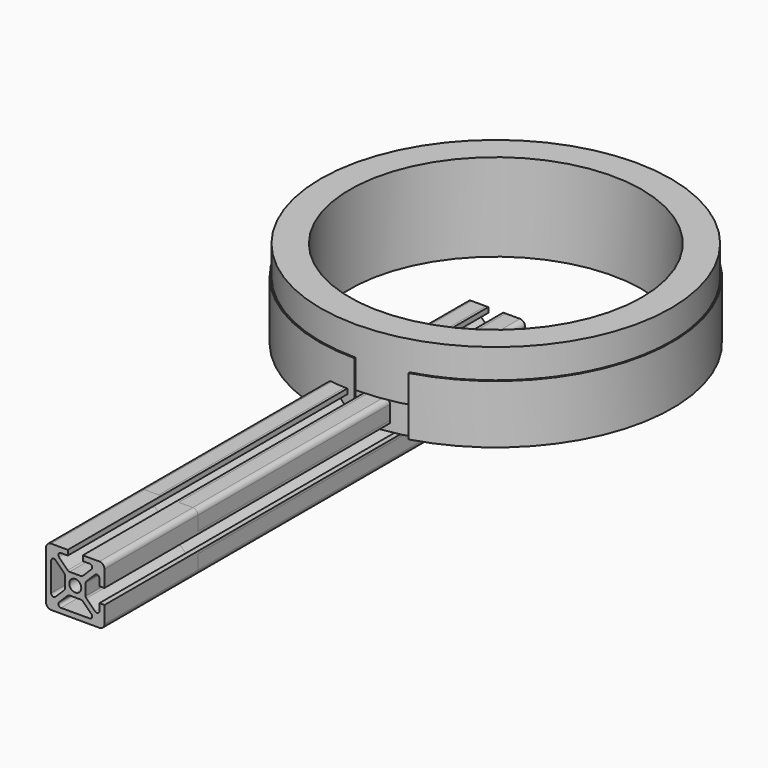
from build123d import *

# Parameters (mm, degrees)
F0_R      = 2.6035
F1_DEPTH  = 228.6
F2_R      = 2.6035
F3_DEPTH  = 177.8
F4_DEPTH  = 228.601
F0_W      = 6.5024
F0_H      = 2.2098
F0_H_2    = 2.1024142881
F0_H_3    = 4.3122142881
F5_DEPTH  = 228.601
F0_W_2    = 4.9525789589
F0_H_4    = 6.5024
F0_W_3    = 2.2098
F0_W_4    = 2.7427789589
F6_DEPTH  = 228.601
F7_R      = 1.10489
F8_R      = 76.2
F8_R_2    = 63.5
F9_DEPTH  = 38.1
F10_R     = 76.2
F10_R_2   = 74.6125
F11_DEPTH = 12.954
F13_DEPTH = 25.4


# Not quite as in the source:
# - a fillet or chamfer is up to 0.001 mm smaller than in the source, because OpenCascade refuses the exact size


with BuildPart() as f1:
    # F0 (on Front) → F1 (new body)
    with BuildSketch(Plane.XZ):
        with BuildLine():
            ThreePointArc((12.7, 10.4902), (12.0527645651, 12.0527645651), (10.4902, 12.7))
            Line((10.4902, 12.7), (3.2512, 12.7))
            Line((3.2512, 12.7), (3.2512, 10.4902))
            Line((3.2512, 10.4902), (6.2601708699, 10.4902))
            ThreePointArc((6.2601708699, 10.4902), (7.2809653653, 9.8081269244), (7.0414531524, 8.6040177175))
            Line((7.0414531524, 8.6040177175), (3.2822531524, 4.8448177175))
            ThreePointArc((3.2822531524, 4.8448177175), (2.9237977943, 4.6053055045), (2.5009708699, 4.5212))
            Line((2.5009708699, 4.5212), (-2.5009708699, 4.5212))
            ThreePointArc((-2.5009708699, 4.5212), (-2.9237977943, 4.6053055045), (-3.2822531524, 4.8448177175))
            Line((-3.2822531524, 4.8448177175), (-7.0414531524, 8.6040177175))
            ThreePointArc((-7.0414531524, 8.6040177175), (-7.2809653653, 9.8081269244), (-6.2601708699, 10.4902))
            Line((-6.2601708699, 10.4902), (-3.2512, 10.4902))
            Line((-3.2512, 10.4902), (-3.2512, 12.7))
            Line((-3.2512, 12.7), (-10.4902, 12.7))
            ThreePointArc((-10.4902, 12.7), (-12.0527645651, 12.0527645651), (-12.7, 10.4902))
            Line((-12.7, 10.4902), (-12.7, -10.4902))
            ThreePointArc((-12.7, -10.4902), (-12.0527645651, -12.0527645651), (-10.4902, -12.7))
            Line((-10.4902, -12.7), (10.4902, -12.7))
            ThreePointArc((10.4902, -12.7), (12.0527645651, -12.0527645651), (12.7, -10.4902))
            Line((12.7, -10.4902), (12.7, -3.2512))
            Line((12.7, -3.2512), (10.4902, -3.2512))
            Line((10.4902, -3.2512), (10.4902, -6.2601708699))
            ThreePointArc((10.4902, -6.2601708699), (9.8081269244, -7.2809653653), (8.6040177175, -7.0414531524))
            Line((8.6040177175, -7.0414531524), (4.8448177175, -3.2822531524))
            ThreePointArc((4.8448177175, -3.2822531524), (4.6053055045, -2.9237977943), (4.5212, -2.5009708699))
            Line((4.5212, -2.5009708699), (4.5212, 2.5009708699))
            ThreePointArc((4.5212, 2.5009708699), (4.6053055045, 2.9237977943), (4.8448177175, 3.2822531524))
            Line((4.8448177175, 3.2822531524), (8.6040177175, 7.0414531524))
            ThreePointArc((8.6040177175, 7.0414531524), (9.8081269244, 7.2809653653), (10.4902, 6.2601708699))
            Line((10.4902, 6.2601708699), (10.4902, 3.2512))
            Line((10.4902, 3.2512), (12.7, 3.2512))
            Line((12.7, 3.2512), (12.7, 10.4902))
        make_face()
        with BuildLine():
            ThreePointArc((7.0414531524, -8.6040177175), (7.2809653653, -9.8081269244), (6.2601708699, -10.4902))
            Line((6.2601708699, -10.4902), (-6.2601708699, -10.4902))
            ThreePointArc((-6.2601708699, -10.4902), (-7.2809653653, -9.8081269244), (-7.0414531524, -8.6040177175))
            Line((-7.0414531524, -8.6040177175), (-3.2822531524, -4.8448177175))
            ThreePointArc((-3.2822531524, -4.8448177175), (-2.9237977943, -4.6053055045), (-2.5009708699, -4.5212))
            Line((-2.5009708699, -4.5212), (2.5009708699, -4.5212))
            ThreePointArc((2.5009708699, -4.5212), (2.9237977943, -4.6053055045), (3.2822531524, -4.8448177175))
            Line((3.2822531524, -4.8448177175), (7.0414531524, -8.6040177175))
        make_face(mode=Mode.SUBTRACT)
        with BuildLine():
            ThreePointArc((-8.6040177175, -7.0414531524), (-9.8081269244, -7.2809653653), (-10.4902, -6.2601708699))
            Line((-10.4902, -6.2601708699), (-10.4902, 6.2601708699))
            ThreePointArc((-10.4902, 6.2601708699), (-9.8081269244, 7.2809653653), (-8.6040177175, 7.0414531524))
            Line((-8.6040177175, 7.0414531524), (-4.8448177175, 3.2822531524))
            ThreePointArc((-4.8448177175, 3.2822531524), (-4.6053055045, 2.9237977943), (-4.5212, 2.5009708699))
            Line((-4.5212, 2.5009708699), (-4.5212, -2.5009708699))
            ThreePointArc((-4.5212, -2.5009708699), (-4.6053055045, -2.9237977943), (-4.8448177175, -3.2822531524))
            Line((-4.8448177175, -3.2822531524), (-8.6040177175, -7.0414531524))
        make_face(mode=Mode.SUBTRACT)
        Circle(F0_R, mode=Mode.SUBTRACT)
    extrude(amount=F1_DEPTH)


with BuildPart() as f3:
    # F2 (on Front) → F3 (new body)
    with BuildSketch(Plane.XZ):
        with BuildLine():
            ThreePointArc((12.7, 10.4902), (12.0527645651, 12.0527645651), (10.4902, 12.7))
            Line((10.4902, 12.7), (-10.4902, 12.7))
            ThreePointArc((-10.4902, 12.7), (-12.0527645651, 12.0527645651), (-12.7, 10.4902))
            Line((-12.7, 10.4902), (-12.7, -10.4902))
            ThreePointArc((-12.7, -10.4902), (-12.0527645651, -12.0527645651), (-10.4902, -12.7))
            Line((-10.4902, -12.7), (10.4902, -12.7))
            ThreePointArc((10.4902, -12.7), (12.0527645651, -12.0527645651), (12.7, -10.4902))
            Line((12.7, -10.4902), (12.7, 10.4902))
        make_face()
        Circle(F2_R, mode=Mode.SUBTRACT)
    extrude(amount=F3_DEPTH)

    # F0 (on Front) → F4 (cut, through all)
    with BuildSketch(Plane.XZ):
        with BuildLine():
            Line((6.2601708699, 10.4902), (3.2512, 10.4902))
            Line((3.2512, 10.4902), (3.2512, 8.3877857119))
            Line((3.2512, 8.3877857119), (-3.2512, 8.3877857119))
            Line((-3.2512, 8.3877857119), (-3.2512, 10.4902))
            Line((-3.2512, 10.4902), (-6.2601708699, 10.4902))
            ThreePointArc((-6.2601708699, 10.4902), (-7.2809653653, 9.8081269244), (-7.0414531524, 8.6040177175))
            Line((-7.0414531524, 8.6040177175), (-3.2822531524, 4.8448177175))
            ThreePointArc((-3.2822531524, 4.8448177175), (-2.9237977943, 4.6053055045), (-2.5009708699, 4.5212))
            Line((-2.5009708699, 4.5212), (2.5009708699, 4.5212))
            ThreePointArc((2.5009708699, 4.5212), (2.9237977943, 4.6053055045), (3.2822531524, 4.8448177175))
            Line((3.2822531524, 4.8448177175), (7.0414531524, 8.6040177175))
            ThreePointArc((7.0414531524, 8.6040177175), (7.2809653653, 9.8081269244), (6.2601708699, 10.4902))
        make_face()
        with BuildLine():
            Line((-10.4902, 6.2601708699), (-10.4902, -6.2601708699))
            ThreePointArc((-10.4902, -6.2601708699), (-9.8081269244, -7.2809653653), (-8.6040177175, -7.0414531524))
            Line((-8.6040177175, -7.0414531524), (-4.8448177175, -3.2822531524))
            ThreePointArc((-4.8448177175, -3.2822531524), (-4.6053055045, -2.9237977943), (-4.5212, -2.5009708699))
            Line((-4.5212, -2.5009708699), (-4.5212, 2.5009708699))
            ThreePointArc((-4.5212, 2.5009708699), (-4.6053055045, 2.9237977943), (-4.8448177175, 3.2822531524))
            Line((-4.8448177175, 3.2822531524), (-8.6040177175, 7.0414531524))
            ThreePointArc((-8.6040177175, 7.0414531524), (-9.8081269244, 7.2809653653), (-10.4902, 6.2601708699))
        make_face()
        with BuildLine():
            Line((7.7474210411, 3.2512), (10.4902, 3.2512))
            Line((10.4902, 3.2512), (10.4902, 6.2601708699))
            ThreePointArc((10.4902, 6.2601708699), (9.8081269244, 7.2809653653), (8.6040177175, 7.0414531524))
            Line((8.6040177175, 7.0414531524), (4.8448177175, 3.2822531524))
            ThreePointArc((4.8448177175, 3.2822531524), (4.6053055045, 2.9237977943), (4.5212, 2.5009708699))
            Line((4.5212, 2.5009708699), (4.5212, -2.5009708699))
            ThreePointArc((4.5212, -2.5009708699), (4.6053055045, -2.9237977943), (4.8448177175, -3.2822531524))
            Line((4.8448177175, -3.2822531524), (8.6040177175, -7.0414531524))
            ThreePointArc((8.6040177175, -7.0414531524), (9.8081269244, -7.2809653653), (10.4902, -6.2601708699))
            Line((10.4902, -6.2601708699), (10.4902, -3.2512))
            Line((10.4902, -3.2512), (7.7474210411, -3.2512))
            Line((7.7474210411, -3.2512), (7.7474210411, 3.2512))
        make_face()
        with BuildLine():
            Line((-6.2601708699, -10.4902), (6.2601708699, -10.4902))
            ThreePointArc((6.2601708699, -10.4902), (7.2809653653, -9.8081269244), (7.0414531524, -8.6040177175))
            Line((7.0414531524, -8.6040177175), (3.2822531524, -4.8448177175))
            ThreePointArc((3.2822531524, -4.8448177175), (2.9237977943, -4.6053055045), (2.5009708699, -4.5212))
            Line((2.5009708699, -4.5212), (-2.5009708699, -4.5212))
            ThreePointArc((-2.5009708699, -4.5212), (-2.9237977943, -4.6053055045), (-3.2822531524, -4.8448177175))
            Line((-3.2822531524, -4.8448177175), (-7.0414531524, -8.6040177175))
            ThreePointArc((-7.0414531524, -8.6040177175), (-7.2809653653, -9.8081269244), (-6.2601708699, -10.4902))
        make_face()
    extrude(amount=F4_DEPTH, mode=Mode.SUBTRACT)

    # F0 (on Front) → F5 (cut, through all)
    with BuildSketch(Plane.XZ):
        with Locations((0, 11.5951)):
            Rectangle(F0_W, F0_H)
        with Locations((0, 9.4389928559)):
            Rectangle(F0_W, F0_H_2)
        with Locations((0, 14.8561071441)):
            Rectangle(F0_W, F0_H_3)
    extrude(amount=F5_DEPTH, mode=Mode.SUBTRACT)

    # F0 (on Front) → F6 (cut, through all)
    with BuildSketch(Plane.XZ):
        with Locations((15.1762894794, 0)):
            Rectangle(F0_W_2, F0_H_4)
        with Locations((11.5951, 0)):
            Rectangle(F0_W_3, F0_H_4)
        with Locations((9.1188105206, 0)):
            Rectangle(F0_W_4, F0_H_4)
    extrude(amount=F6_DEPTH, mode=Mode.SUBTRACT)

    # F7 (radius 1.1049 in the source; OpenCascade refuses exactly that, so slightly less here)
    f7_edges = [f3.edges().sort_by_distance(p)[0] for p in [
        (-3.2512, -88.9, 12.7),
        (-3.2512, -88.9, 10.4902),
        (3.2512, -88.9, 12.7),
        (12.7, -88.9, 3.2512),
        (12.7, -88.9, -3.2512),
        (10.4902, -88.9, -3.2512),
        (3.2512, -88.9, 10.4902),
        (10.4902, -88.9, 3.2512),
    ]]
    fillet(f7_edges, radius=F7_R)


with BuildPart() as f9:
    # F8 (on Top) → F9 (new body)
    with BuildSketch(Plane.XY):
        Circle(F8_R)
        Circle(F8_R_2, mode=Mode.SUBTRACT)
    extrude(amount=F9_DEPTH)

    # F10 (on Top) → F11 (cut)
    with BuildSketch(Plane.XY):
        Circle(F10_R)
        Circle(F10_R_2, mode=Mode.SUBTRACT)
    extrude(amount=F11_DEPTH, mode=Mode.SUBTRACT)


with BuildPart() as f13:
    # F12 (on Top) → F13 (new body)
    with BuildSketch(Plane.XY):
        with BuildLine():
            ThreePointArc((0, -76.2), (-10.6049902932, 75.4584268381), (21.0035665133, -73.2481412305))
            Line((21.0035665133, -73.2481412305), (21.1785962342, -73.8585424074))
            ThreePointArc((21.1785962342, -73.8585424074), (-10.6933652123, 76.0872470618), (0, -76.835))
            Line((0, -76.835), (0, -76.2))
        make_face()
    extrude(amount=F13_DEPTH)


solid = Compound([f1.part, f3.part, f9.part, f13.part])
